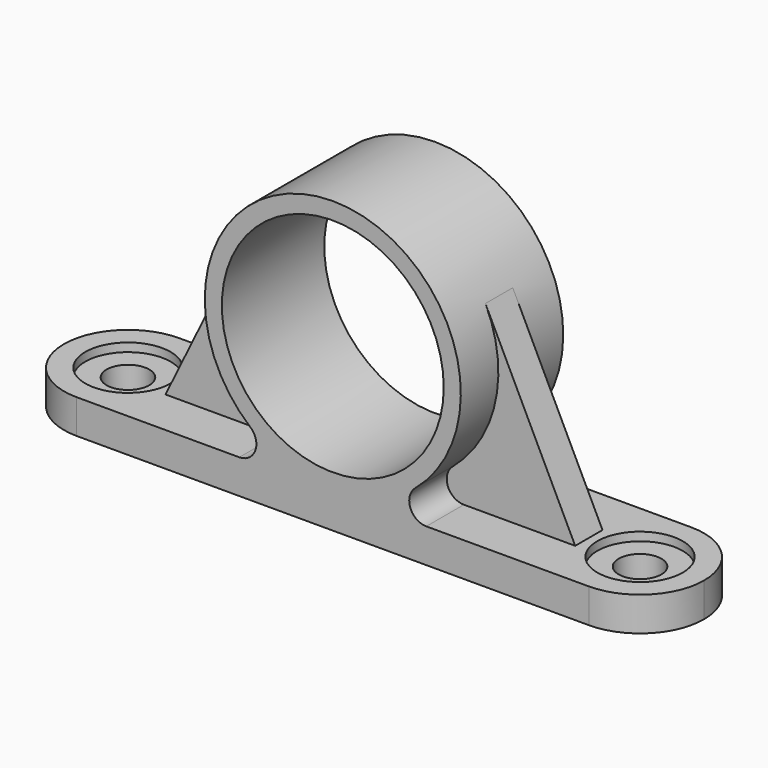
from build123d import *

# Parameters (mm, degrees)
F2_DEPTH       = 7.5
F3_R           = 13
F4_DEPTH       = 15.001
F5_R           = 7.49999
F7_D           = 5
F7_CBORE_D     = 10
F7_CBORE_DEPTH = 1
F9_DEPTH       = 2


# Not quite as in the source:
# - a fillet or chamfer is up to 0.001 mm smaller than in the source, because OpenCascade refuses the exact size


with BuildPart() as f2:
    # F1 (on Front) → F2 (new body, symmetric)
    with BuildSketch(Plane.XZ):
        with BuildLine():
            Line((-37.5, 0), (0, 0))
            Line((0, 0), (37.5, 0))
            Line((37.5, 0), (37.5, 4))
            Line((37.5, 4), (10.9544511501, 4))
            ThreePointArc((10.9544511501, 4), (9.0757782768, 5.3140056594), (9.6656921913, 7.5294117647))
            ThreePointArc((9.6656921913, 7.5294117647), (14.0900465494, 24.1449575543), (0, 34))
            ThreePointArc((0, 34), (-14.0900465494, 24.1449575543), (-9.6656921913, 7.5294117647))
            ThreePointArc((-9.6656921913, 7.5294117647), (-9.0757782768, 5.3140056594), (-10.9544511501, 4))
            Line((-10.9544511501, 4), (-37.5, 4))
            Line((-37.5, 4), (-37.5, 0))
        make_face()
    extrude(amount=F2_DEPTH, both=True)

    # F3 (on face) → F4 (cut, through all)
    with BuildSketch(Plane.XZ.offset(7.5)):
        with Locations((0, 19)):
            Circle(F3_R)
    extrude(amount=-F4_DEPTH, mode=Mode.SUBTRACT)

    # F5 (radius 7.5 in the source; OpenCascade refuses exactly that, so slightly less here)
    f5_edges = [f2.edges().sort_by_distance(p)[0] for p in [
        (37.5, -7.5, 2),
        (37.5, 7.5, 2),
        (-37.5, -7.5, 2),
        (-37.5, 7.5, 2),
    ]]
    fillet(f5_edges, radius=F5_R)

    # F7 (through all)
    with Locations(Plane.XY.offset(4)):
        with Locations((30, 0), (-30, 0)):
            CounterBoreHole(F7_D / 2, F7_CBORE_D / 2, F7_CBORE_DEPTH)

    # F8 (on Front) → F9 (join, symmetric)
    with BuildSketch(Plane.XZ):
        with BuildLine():
            Line((10.9544511501, 4), (24, 4))
            Line((24, 4), (13.4831460674, 25.5730337079))
            ThreePointArc((13.4831460674, 25.5730337079), (14.6751576274, 15.8952055444), (9.6656921913, 7.5294117647))
            ThreePointArc((9.6656921913, 7.5294117647), (9.0757782768, 5.3140056594), (10.9544511501, 4))
        make_face()
    extrude(amount=F9_DEPTH, both=True)

    # F10: F2 across plane


with BuildPart() as f2_1:
    add(f2.part)
    add(f2.part.mirror(Plane.YZ))


solid = f2_1.part
